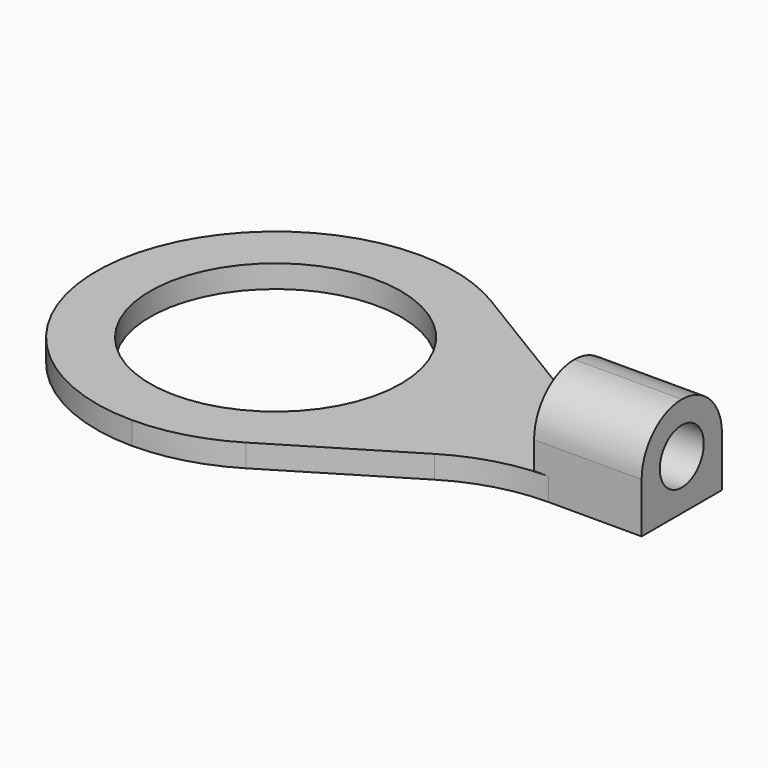
from build123d import *

# Parameters (mm, degrees)
F0_R     = 5.25
F1_DEPTH = 0.95
F3_DEPTH = 3.25
F4_R     = 2.09999
F5_R     = 1.15
F6_DEPTH = 25


# Not quite as in the source:
# - a fillet or chamfer is up to 0.001 mm smaller than in the source, because OpenCascade refuses the exact size


with BuildPart() as f1:
    # F0 (on Top) → F1 (new body)
    with BuildSketch(Plane.XY):
        with BuildLine():
            Line((20.596680348, 5.4), (24.5, 5.4))
            Line((24.5, 5.4), (24.5, 9.6))
            Line((24.5, 9.6), (20.596680348, 9.6))
            ThreePointArc((20.596680348, 9.6), (18.5774207214, 9.8769403602), (16.7072849584, 10.6873091839))
            Line((16.7072849584, 10.6873091839), (11.3893953897, 13.9126908161))
            ThreePointArc((11.3893953897, 13.9126908161), (9.5192596266, 14.7230596398), (7.5, 15))
            ThreePointArc((7.5, 15), (2.1966991411, 12.8033008589), (0, 7.5))
            ThreePointArc((0, 7.5), (2.1966991411, 2.1966991411), (7.5, 0))
            ThreePointArc((7.5, 0), (9.5192596266, 0.2769403602), (11.3893953897, 1.0873091839))
            Line((11.3893953897, 1.0873091839), (16.7072849584, 4.3126908161))
            ThreePointArc((16.7072849584, 4.3126908161), (18.5774207214, 5.1230596398), (20.596680348, 5.4))
        make_face()
        with Locations((7.5, 7.5)):
            Circle(F0_R, mode=Mode.SUBTRACT)
    extrude(amount=F1_DEPTH)

    # F2 (on face) → F3 (join)
    with BuildSketch(Plane.XY.offset(0.95)):
        Polygon((24.5, 5.4), (24.5, 9.6), (20.596680348, 9.6), (20, 9.6), (20, 5.4), (20.596680348, 5.4), align=None)
    extrude(amount=F3_DEPTH)

    # F4 (radius 2.1 in the source; OpenCascade refuses exactly that, so slightly less here)
    f4_edges = [f1.edges().sort_by_distance(p)[0] for p in [
        (22.25, 9.6, 4.2),
        (22.25, 5.4, 4.2),
    ]]
    fillet(f4_edges, radius=F4_R)

    # F5 (on face) → F6 (cut)
    with BuildSketch(Plane.YZ.offset(24.5)):
        with Locations((7.5, 2.1)):
            Circle(F5_R)
    extrude(amount=-F6_DEPTH, mode=Mode.SUBTRACT)


solid = f1.part
